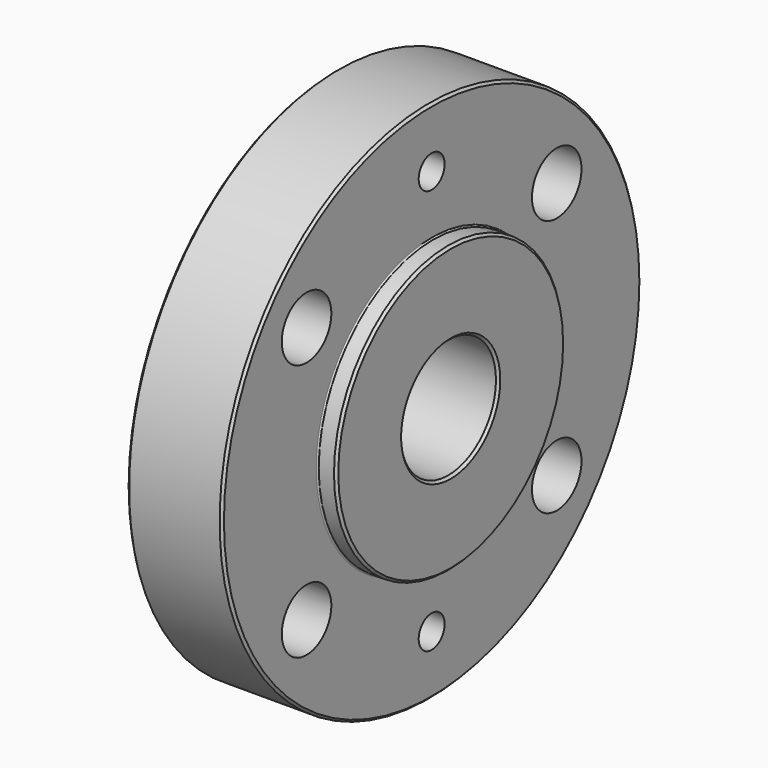
from build123d import *

# Parameters (mm, degrees)
F0_R           = 55
F0_R_2         = 30
F0_R_3         = 21
F0_R_4         = 12.5
F1_DEPTH       = 20
F2_DEPTH       = 1.6
F3_R           = 30
F3_R_2         = 12.5
F4_DEPTH       = 4
F5_D           = 5
F5_DEPTH       = 12
F5_CBORE_D     = 6
F5_CBORE_DEPTH = 1
F5_TIP         = 1.5021515476
F6_D           = 13
F6_CBORE_D     = 20
F6_CBORE_DEPTH = 10
F7_D           = 6.8
F7_CBORE_D     = 8
F7_CBORE_DEPTH = 1.2
F8_SIZE2       = 0.5
F8_SIZE        = 0.5
F9_R           = 0.3


with BuildPart() as f1:
    # F0 (on Right) → F1 (new body)
    with BuildSketch(Plane.YZ):
        Circle(F0_R)
        Circle(F0_R_2, mode=Mode.SUBTRACT)
        Circle(F0_R_2)
        Circle(F0_R_3, mode=Mode.SUBTRACT)
        Circle(F0_R_3)
        Circle(F0_R_4, mode=Mode.SUBTRACT)
    extrude(amount=F1_DEPTH)

    # F0 (on Right) → F2 (join)
    with BuildSketch(Plane.YZ):
        Circle(F0_R_3)
        Circle(F0_R_4, mode=Mode.SUBTRACT)
    extrude(amount=-F2_DEPTH)

    # F3 (on face) → F4 (join)
    with BuildSketch(Plane.YZ.offset(20)):
        Circle(F3_R)
        Circle(F3_R_2, mode=Mode.SUBTRACT)
    extrude(amount=F4_DEPTH)

    # F5
    with Locations(Plane(origin=(0, 0, 0), x_dir=(0, 1, 0), z_dir=(-1, 0, 0))):
        with Locations((-15.5, -26.8467875173), (-31, 0), (-15.5, 26.8467875173), (15.5, -26.8467875173), (31, 0), (15.5, 26.8467875173)):
            CounterBoreHole(F5_D / 2, F5_CBORE_D / 2, F5_CBORE_DEPTH, depth=F5_DEPTH)
            with Locations((0, 0, -(F5_DEPTH + F5_TIP / 2))):  # 118° drill point
                Cone(0, F5_D / 2, F5_TIP, mode=Mode.SUBTRACT)

    # F6 (through all)
    with Locations(Plane(origin=(0, 0, 0), x_dir=(0, 1, 0), z_dir=(-1, 0, 0))):
        with Locations((-32.8214868646, 27), (-32.8214868646, -27), (32.8214868646, -27), (32.8214868646, 27)):
            CounterBoreHole(F6_D / 2, F6_CBORE_D / 2, F6_CBORE_DEPTH)

    # F7 (through all)
    with Locations(Plane(origin=(0, 0, 0), x_dir=(0, 1, 0), z_dir=(-1, 0, 0))):
        with Locations((0, -42.5), (0, 42.5)):
            CounterBoreHole(F7_D / 2, F7_CBORE_D / 2, F7_CBORE_DEPTH)

    # F8
    f8_edges = [f1.edges().sort_by_distance(p)[0] for p in [
        (20, -55, 0),
        (0, -55, 0),
        (24, -30, 0),
        (24, -12.5, 0),
        (-1.6, -12.5, 0),
    ]]
    chamfer(f8_edges, length=F8_SIZE, length2=F8_SIZE2)

    # F9
    f9_edges = [f1.edges().sort_by_distance(p)[0] for p in [
        (20, -30, 0),
        (0, -21, 0),
        (-1.6, -21, 0),
    ]]
    fillet(f9_edges, radius=F9_R)


solid = f1.part
